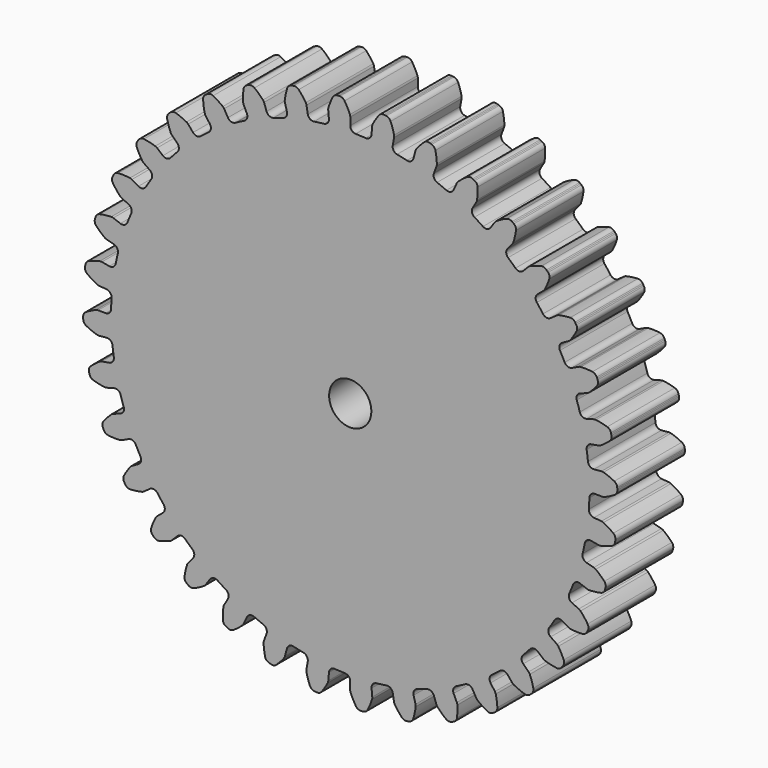
from build123d import *

# Parameters (mm, degrees)
F1_DEPTH = 12.7
F2_R     = 3.175
F3_DEPTH = 12.701


# Not quite as in the source:
# - ends of sketch curves that miss each other by under 0.0002 mm in the source are joined


with BuildPart() as f1:
    # F0 (on Front) → F1 (new body)
    with BuildSketch(Plane.XZ):
        with BuildLine():
            ThreePointArc((-3.2109370393, 36.662551447), (-3.393615267, 36.0650718095), (-3.9425466273, 35.7666968543))
            ThreePointArc((-3.9425466273, 35.7666968543), (-4.6967674834, 35.6754909284), (-5.4488947177, 35.568382366))
            ThreePointArc((-5.4488947177, 35.568382366), (-6.0563468164, 35.7145165506), (-6.3874395437, 36.2443569587))
            Line((-6.3874395437, 36.2443569587), (-6.5805401603, 37.3664180659))
            ThreePointArc((-6.5805401603, 37.3664180659), (-6.6228583498, 37.5208029851), (-6.6941779071, 37.6641175104))
            ThreePointArc((-6.6941779071, 37.6641175104), (-7.1901089353, 38.3817855666), (-7.7496189767, 39.0510714078))
            ThreePointArc((-7.7496189767, 39.0510714078), (-8.1067459622, 39.2794815465), (-8.5301465281, 39.3005252169))
            Line((-8.5301465281, 39.3005252169), (-8.7037167329, 39.2635272434))
            Line((-8.7037167329, 39.2635272434), (-8.7052373822, 39.2631901235))
            Line((-8.7052373822, 39.2631901235), (-8.8781814297, 39.2233677368))
            ThreePointArc((-8.8781814297, 39.2233677368), (-9.2530192202, 39.0253588833), (-9.4801558924, 38.6674206101))
            ThreePointArc((-9.4801558924, 38.6674206101), (-9.704391781, 37.8243824794), (-9.8505583073, 36.9643648225))
            ThreePointArc((-9.8505583073, 36.9643648225), (-9.8546284418, 36.8043368048), (-9.8277358603, 36.6465321107))
            Line((-9.8277358603, 36.6465321107), (-9.5285409381, 35.5479915448))
            ThreePointArc((-9.5285409381, 35.5479915448), (-9.6046926228, 34.9278672241), (-10.0934722151, 34.5387043246))
            ThreePointArc((-10.0934722151, 34.5387043246), (-10.8203970188, 34.3179149444), (-11.5424985437, 34.0818280781))
            ThreePointArc((-11.5424985437, 34.0818280781), (-12.166098015, 34.1202592061), (-12.5841665211, 34.5845564992))
            Line((-12.5841665211, 34.5845564992), (-12.9691773719, 35.6560394067))
            ThreePointArc((-12.9691773719, 35.6560394067), (-13.037661313, 35.8007303955), (-13.1327836721, 35.9294831401))
            ThreePointArc((-13.1327836721, 35.9294831401), (-13.7458021437, 36.5501306866), (-14.413032237, 37.1120906729))
            ThreePointArc((-14.413032237, 37.1120906729), (-14.8043966655, 37.2750162981), (-15.2250190205, 37.2222175312))
            Line((-15.2250190205, 37.2222175312), (-15.3895276731, 37.1556414903))
            Line((-15.3895276731, 37.1556414903), (-15.3909666802, 37.1550454341))
            Line((-15.3909666802, 37.1550454341), (-15.5543682341, 37.0857966202))
            ThreePointArc((-15.5543682341, 37.0857966202), (-15.8891275197, 36.8257060668), (-16.0506581466, 36.4337638111))
            ThreePointArc((-16.0506581466, 36.4337638111), (-16.1250953531, 35.5645951705), (-16.1197007825, 34.6922615633))
            ThreePointArc((-16.1197007825, 34.6922615633), (-16.0959205089, 34.5339579593), (-16.0420339886, 34.3832205209))
            Line((-16.0420339886, 34.3832205209), (-15.5566249422, 33.3533239076))
            ThreePointArc((-15.5566249422, 33.3533239076), (-15.5239362535, 32.7293970675), (-15.9377127572, 32.2612707414))
            ThreePointArc((-15.9377127572, 32.2612707414), (-16.6152542662, 31.9176064805), (-17.2853893923, 31.5597146903))
            ThreePointArc((-17.2853893923, 31.5597146903), (-17.9061884817, 31.4892750513), (-18.3985299667, 31.873921791))
            Line((-18.3985299667, 31.873921791), (-18.9637526919, 32.862270033))
            ThreePointArc((-18.9637526919, 32.862270033), (-19.0563215345, 32.992870729), (-19.1723564507, 33.1031496058))
            ThreePointArc((-19.1723564507, 33.1031496058), (-19.8838361097, 33.607918581), (-20.6385128062, 34.0454778426))
            ThreePointArc((-20.6385128062, 34.0454778426), (-21.0522232676, 34.1379685416), (-21.4572870141, 34.0129316012))
            Line((-21.4572870141, 34.0129316012), (-21.6077356025, 33.9188003722))
            Line((-21.6077356025, 33.9188003722), (-21.6090492437, 33.9179634904))
            Line((-21.6090492437, 33.9179634904), (-21.7579434305, 33.8213923396))
            ThreePointArc((-21.7579434305, 33.8213923396), (-22.0424527198, 33.5071228062), (-22.1334692751, 33.0930855351))
            ThreePointArc((-22.1334692751, 33.0930855351), (-22.0558460626, 32.2241956338), (-21.8990543065, 31.3660514916))
            ThreePointArc((-21.8990543065, 31.3660514916), (-21.8481461763, 31.2142822763), (-21.7689030319, 31.0751921743))
            Line((-21.7689030319, 31.0751921743), (-21.1120287695, 30.145232401))
            ThreePointArc((-21.1120287695, 30.145232401), (-20.9714929366, 29.5364607428), (-21.297693962, 29.0035947717))
            ThreePointArc((-21.297693962, 29.0035947717), (-21.9052654205, 28.5474976948), (-22.5030724311, 28.0786753416))
            ThreePointArc((-22.5030724311, 28.0786753416), (-23.1022084724, 27.9015052085), (-23.6538633894, 28.1948140982))
            Line((-23.6538633894, 28.1948140982), (-24.3821239824, 29.0699972134))
            ThreePointArc((-24.3821239824, 29.0699972134), (-24.4959650692, 29.1825393805), (-24.6293868802, 29.2709936216))
            ThreePointArc((-24.6293868802, 29.2709936216), (-25.4177097773, 29.6445468757), (-26.2369026074, 29.9444103958))
            ThreePointArc((-26.2369026074, 29.9444103958), (-26.6603887185, 29.9636558856), (-27.0375861998, 29.7701799558))
            Line((-27.0375861998, 29.7701799558), (-27.1694034197, 29.6513536685))
            Line((-27.1694034197, 29.6513536685), (-27.1705517807, 29.6503013895))
            Line((-27.1705517807, 29.6503013895), (-27.3004145259, 29.5293421672))
            ThreePointArc((-27.3004145259, 29.5293421672), (-27.526029148, 29.1704425746), (-27.5437661397, 28.746890601))
            ThreePointArc((-27.5437661397, 28.746890601), (-27.3164410503, 27.9046802191), (-27.0130161468, 27.0867998174))
            ThreePointArc((-27.0130161468, 27.0867998174), (-26.9365269778, 26.9461764215), (-26.8343349721, 26.8229598383))
            Line((-26.8343349721, 26.8229598383), (-26.0259542858, 26.0211932622))
            ThreePointArc((-26.0259542858, 26.0211932622), (-25.7818414189, 25.4460740047), (-26.0105555129, 24.8646592514))
            ThreePointArc((-26.0105555129, 24.8646592514), (-26.5296961696, 24.3099876374), (-27.0370110011, 23.7444796512))
            ThreePointArc((-27.0370110011, 23.7444796512), (-27.596279549, 23.4659622487), (-28.1904861423, 23.6590212463))
            Line((-28.1904861423, 23.6590212463), (-29.0596567737, 24.3944472386))
            ThreePointArc((-29.0596567737, 24.3944472386), (-29.1913111008, 24.4855113401), (-29.3380658525, 24.5494533081))
            ThreePointArc((-29.3380658525, 24.5494533081), (-30.1792791952, 24.7804406144), (-31.0380973993, 24.9334971918))
            ThreePointArc((-31.0380973993, 24.9334971918), (-31.4584917491, 24.8789127079), (-31.7963620104, 24.622876457))
            Line((-31.7963620104, 24.622876457), (-31.9055426623, 24.4829655879))
            Line((-31.9055426623, 24.4829655879), (-31.9064908509, 24.4817298846))
            Line((-31.9064908509, 24.4817298846), (-32.0133763406, 24.3400578756))
            ThreePointArc((-32.0133763406, 24.3400578756), (-32.1732411094, 23.9474332063), (-32.117159608, 23.5272359426))
            ThreePointArc((-32.117159608, 23.5272359426), (-31.7470397994, 22.7372952164), (-31.3062011607, 21.9845294373))
            ThreePointArc((-31.3062011607, 21.9845294373), (-31.2064550377, 21.8593246316), (-31.084419223, 21.7557254407))
            Line((-31.084419223, 21.7557254407), (-30.1490943509, 21.1065133335))
            ThreePointArc((-30.1490943509, 21.1065133335), (-29.808821696, 20.5825211842), (-29.9330994966, 19.9702236418))
            ThreePointArc((-29.9330994966, 19.9702236418), (-30.3480355252, 19.333830907), (-30.7494436732, 18.6888199618))
            ThreePointArc((-30.7494436732, 18.6888199618), (-31.2518516358, 18.3174179003), (-31.870555239, 18.4043610059))
            Line((-31.870555239, 18.4043610059), (-32.8542265987, 18.9776843286))
            ThreePointArc((-32.8542265987, 18.9776843286), (-32.9996939161, 19.0445034278), (-33.1553225396, 19.0819902785))
            ThreePointArc((-33.1553225396, 19.0819902785), (-34.0238664862, 19.1633932046), (-34.8962153078, 19.1649922926))
            ThreePointArc((-34.8962153078, 19.1649922926), (-35.3007444267, 19.0382363568), (-35.5890214511, 18.7274193167))
            Line((-35.5890214511, 18.7274193167), (-35.6722481362, 18.5706749869))
            Line((-35.6722481362, 18.5706749869), (-35.6729673419, 18.5692934055))
            Line((-35.6729673419, 18.5692934055), (-35.7536279147, 18.4112132422))
            ThreePointArc((-35.7536279147, 18.4112132422), (-35.8428854202, 17.9967931981), (-35.7146894336, 17.5927181255))
            ThreePointArc((-35.7146894336, 17.5927181255), (-35.2130208091, 16.8790490041), (-34.6481630941, 16.2142702549))
            ThreePointArc((-34.6481630941, 16.2142702549), (-34.5281907524, 16.108288324), (-34.3900191252, 16.0274543345))
            Line((-34.3900191252, 16.0274543345), (-33.3561694403, 15.5505226775))
            ThreePointArc((-33.3561694403, 15.5505226775), (-32.9300760098, 15.0935788729), (-32.9461413989, 14.4690028923))
            ThreePointArc((-32.9461413989, 14.4690028923), (-33.2442651782, 13.7702255079), (-33.5275700593, 13.0653099349))
            ThreePointArc((-33.5275700593, 13.0653099349), (-33.9578520249, 12.6123080781), (-34.5822536419, 12.5904935694))
            Line((-34.5822536419, 12.5904935694), (-35.6505373737, 12.9842940835))
            ThreePointArc((-35.6505373737, 12.9842940835), (-35.8053977304, 13.0248379159), (-35.9651715287, 13.0347306302))
            ThreePointArc((-35.9651715287, 13.0347306302), (-36.834655811, 12.9640757894), (-37.6940293725, 12.8141688005))
            ThreePointArc((-37.6940293725, 12.8141688005), (-38.0704018478, 12.6190928279), (-38.3003264839, 12.2629390171))
            Line((-38.3003264839, 12.2629390171), (-38.3550704014, 12.0941238237))
            Line((-38.3550704014, 12.0941238237), (-38.3555387717, 12.0926383428))
            Line((-38.3555387717, 12.0926383428), (-38.4075235969, 11.9229532109))
            ThreePointArc((-38.4075235969, 11.9229532109), (-38.4234617948, 11.4993297353), (-38.2270464933, 11.1236544704))
            ThreePointArc((-38.2270464933, 11.1236544704), (-37.609072, 10.5079414291), (-36.9373581246, 9.9513486757))
            ThreePointArc((-36.9373581246, 9.9513486757), (-36.8008048633, 9.867809827), (-36.6506956986, 9.8121971386))
            Line((-36.6506956986, 9.8121971386), (-35.5497342003, 9.522037259))
            ThreePointArc((-35.5497342003, 9.522037259), (-35.0507666275, 9.1460258052), (-34.9581314664, 8.5281488117))
            ThreePointArc((-34.9581314664, 8.5281488117), (-35.1303846562, 7.7882187749), (-35.2869781949, 7.044817077))
            ThreePointArc((-35.2869781949, 7.044817077), (-35.6320602637, 6.5239796571), (-36.2431877675, 6.3940703568))
            Line((-36.2431877675, 6.3940703568), (-37.3636246105, 6.5963826331))
            ThreePointArc((-37.3636246105, 6.5963826331), (-37.5231726531, 6.6094192948), (-37.6822369802, 6.5914172876))
            ThreePointArc((-37.6822369802, 6.5914172876), (-38.5262427581, 6.3708514914), (-39.3465294288, 6.0739932736))
            ThreePointArc((-39.3465294288, 6.0739932736), (-39.6833093734, 5.816524549), (-39.8478954775, 5.4258555208))
            Line((-39.8478954775, 5.4258555208), (-39.8724932611, 5.2500988279))
            Line((-39.8724932611, 5.2500988279), (-39.8726965647, 5.2485545832))
            Line((-39.8726965647, 5.2485545832), (-39.8944261097, 5.0724202796))
            ThreePointArc((-39.8944261097, 5.0724202796), (-39.836560726, 4.6524649574), (-39.5778940892, 4.3166042031))
            ThreePointArc((-39.5778940892, 4.3166042031), (-38.8623905695, 3.817555371), (-38.1042302198, 3.3860604026))
            ThreePointArc((-38.1042302198, 3.3860604026), (-37.9552451405, 3.3275029217), (-37.7977594293, 3.2988012979))
            Line((-37.7977594293, 3.2988012979), (-36.6631382757, 3.2042295567))
            ThreePointArc((-36.6631382757, 3.2042295567), (-36.1064574377, 2.9205753715), (-35.907936399, 2.3281712448))
            ThreePointArc((-35.907936399, 2.3281712448), (-35.9490851733, 1.5695709554), (-35.9742093542, 0.8102710171))
            ThreePointArc((-35.9742093542, 0.8102710171), (-36.2236063821, 0.2374234155), (-36.8028909726, 0.003366552))
            Line((-36.8028909726, 0.003366552), (-37.9414370205, 0.0080434342))
            ThreePointArc((-37.9414370205, 0.0080434342), (-38.1008249623, -0.0068231871), (-38.2543467292, -0.0521729338))
            ThreePointArc((-38.2543467292, -0.0521729338), (-39.0472293143, -0.4159479052), (-39.8035050988, -0.8507374652))
            ThreePointArc((-39.8035050988, -0.8507374652), (-40.0904596244, -1.162775885), (-40.1847063309, -1.5760898499))
            Line((-40.1847063309, -1.5760898499), (-40.1784105895, -1.753447764))
            Line((-40.1784105895, -1.753447764), (-40.1783426492, -1.7550038515))
            Line((-40.1783426492, -1.7550038515), (-40.1691566727, -1.9322355751))
            ThreePointArc((-40.1691566727, -1.9322355751), (-40.0392459178, -2.3357626139), (-39.7261874005, -2.6216038985))
            ThreePointArc((-39.7261874005, -2.6216038985), (-38.9348950667, -2.9888251752), (-38.1133245614, -3.2821116025))
            ThreePointArc((-38.1133245614, -3.2821116025), (-37.9564345003, -3.3139084761), (-37.7963573663, -3.314826951))
            Line((-37.7963573663, -3.314826951), (-36.662551447, -3.2109370393))
            ThreePointArc((-36.662551447, -3.2109370393), (-36.0650718095, -3.393615267), (-35.7666968543, -3.9425466273))
            ThreePointArc((-35.7666968543, -3.9425466273), (-35.6754909284, -4.6967674834), (-35.568382366, -5.4488947177))
            ThreePointArc((-35.568382366, -5.4488947177), (-35.7145165506, -6.0563468164), (-36.2443569587, -6.3874395437))
            Line((-36.2443569587, -6.3874395437), (-37.3664180659, -6.5805401603))
            ThreePointArc((-37.3664180659, -6.5805401603), (-37.5208029851, -6.6228583498), (-37.6641175104, -6.6941779071))
            ThreePointArc((-37.6641175104, -6.6941779071), (-38.3817855666, -7.1901089353), (-39.0510714078, -7.7496189767))
            ThreePointArc((-39.0510714078, -7.7496189767), (-39.2794815465, -8.1067459622), (-39.3005252169, -8.5301465281))
            Line((-39.3005252169, -8.5301465281), (-39.2635272434, -8.7037167329))
            Line((-39.2635272434, -8.7037167329), (-39.2631901235, -8.7052373822))
            Line((-39.2631901235, -8.7052373822), (-39.2233677368, -8.8781814297))
            ThreePointArc((-39.2233677368, -8.8781814297), (-39.0253588833, -9.2530192202), (-38.6674206101, -9.4801558924))
            ThreePointArc((-38.6674206101, -9.4801558924), (-37.8243824794, -9.704391781), (-36.9643648225, -9.8505583073))
            ThreePointArc((-36.9643648225, -9.8505583073), (-36.8043368048, -9.8546284418), (-36.6465321107, -9.8277358603))
            Line((-36.6465321107, -9.8277358603), (-35.5479915448, -9.5285409381))
            ThreePointArc((-35.5479915448, -9.5285409381), (-34.9278672241, -9.6046926228), (-34.5387043246, -10.0934722151))
            ThreePointArc((-34.5387043246, -10.0934722151), (-34.3179149444, -10.8203970188), (-34.0818280781, -11.5424985437))
            ThreePointArc((-34.0818280781, -11.5424985437), (-34.1202592061, -12.166098015), (-34.5845564992, -12.5841665211))
            Line((-34.5845564992, -12.5841665211), (-35.6560394067, -12.9691773719))
            ThreePointArc((-35.6560394067, -12.9691773719), (-35.8007303955, -13.037661313), (-35.9294831401, -13.1327836721))
            ThreePointArc((-35.9294831401, -13.1327836721), (-36.5501306866, -13.7458021437), (-37.1120906729, -14.413032237))
            ThreePointArc((-37.1120906729, -14.413032237), (-37.2750162981, -14.8043966655), (-37.2222175312, -15.2250190205))
            Line((-37.2222175312, -15.2250190205), (-37.1556414903, -15.3895276731))
            Line((-37.1556414903, -15.3895276731), (-37.1550454341, -15.3909666802))
            Line((-37.1550454341, -15.3909666802), (-37.0857966202, -15.5543682341))
            ThreePointArc((-37.0857966202, -15.5543682341), (-36.8257060668, -15.8891275197), (-36.4337638111, -16.0506581466))
            ThreePointArc((-36.4337638111, -16.0506581466), (-35.5645951705, -16.1250953531), (-34.6922615633, -16.1197007825))
            ThreePointArc((-34.6922615633, -16.1197007825), (-34.5339579593, -16.0959205089), (-34.3832205209, -16.0420339886))
            Line((-34.3832205209, -16.0420339886), (-33.3533239076, -15.5566249422))
            ThreePointArc((-33.3533239076, -15.5566249422), (-32.7293970675, -15.5239362535), (-32.2612707414, -15.9377127572))
            ThreePointArc((-32.2612707414, -15.9377127572), (-31.9176064805, -16.6152542662), (-31.5597146903, -17.2853893923))
            ThreePointArc((-31.5597146903, -17.2853893923), (-31.4892750513, -17.9061884817), (-31.873921791, -18.3985299667))
            Line((-31.873921791, -18.3985299667), (-32.862270033, -18.9637526919))
            ThreePointArc((-32.862270033, -18.9637526919), (-32.992870729, -19.0563215345), (-33.1031496058, -19.1723564507))
            ThreePointArc((-33.1031496058, -19.1723564507), (-33.607918581, -19.8838361097), (-34.0454778426, -20.6385128062))
            ThreePointArc((-34.0454778426, -20.6385128062), (-34.1379685416, -21.0522232676), (-34.0129316012, -21.4572870141))
            Line((-34.0129316012, -21.4572870141), (-33.9188003722, -21.6077356025))
            Line((-33.9188003722, -21.6077356025), (-33.9179634904, -21.6090492437))
            Line((-33.9179634904, -21.6090492437), (-33.8213923396, -21.7579434305))
            ThreePointArc((-33.8213923396, -21.7579434305), (-33.5071228062, -22.0424527198), (-33.0930855351, -22.1334692751))
            ThreePointArc((-33.0930855351, -22.1334692751), (-32.2241956338, -22.0558460626), (-31.3660514916, -21.8990543065))
            ThreePointArc((-31.3660514916, -21.8990543065), (-31.2142822763, -21.8481461763), (-31.0751921743, -21.7689030319))
            Line((-31.0751921743, -21.7689030319), (-30.145232401, -21.1120287695))
            ThreePointArc((-30.145232401, -21.1120287695), (-29.5364607428, -20.9714929366), (-29.0035947717, -21.297693962))
            ThreePointArc((-29.0035947717, -21.297693962), (-28.5474976948, -21.9052654205), (-28.0786753416, -22.5030724311))
            ThreePointArc((-28.0786753416, -22.5030724311), (-27.9015052085, -23.1022084724), (-28.1948140982, -23.6538633894))
            Line((-28.1948140982, -23.6538633894), (-29.0699972134, -24.3821239824))
            ThreePointArc((-29.0699972134, -24.3821239824), (-29.1825393805, -24.4959650692), (-29.2709936216, -24.6293868802))
            ThreePointArc((-29.2709936216, -24.6293868802), (-29.6445468757, -25.4177097773), (-29.9444103958, -26.2369026074))
            ThreePointArc((-29.9444103958, -26.2369026074), (-29.9636558856, -26.6603887185), (-29.7701799558, -27.0375861998))
            Line((-29.7701799558, -27.0375861998), (-29.6513536685, -27.1694034197))
            Line((-29.6513536685, -27.1694034197), (-29.6503013895, -27.1705517807))
            Line((-29.6503013895, -27.1705517807), (-29.5293421672, -27.3004145259))
            ThreePointArc((-29.5293421672, -27.3004145259), (-29.1704425746, -27.526029148), (-28.746890601, -27.5437661397))
            ThreePointArc((-28.746890601, -27.5437661397), (-27.9046802191, -27.3164410503), (-27.0867998174, -27.0130161468))
            ThreePointArc((-27.0867998174, -27.0130161468), (-26.9461764215, -26.9365269778), (-26.8229598383, -26.8343349721))
            Line((-26.8229598383, -26.8343349721), (-26.0211932622, -26.0259542858))
            ThreePointArc((-26.0211932622, -26.0259542858), (-25.4460740047, -25.7818414189), (-24.8646592514, -26.0105555129))
            ThreePointArc((-24.8646592514, -26.0105555129), (-24.3099876374, -26.5296961696), (-23.7444796512, -27.0370110011))
            ThreePointArc((-23.7444796512, -27.0370110011), (-23.4659622487, -27.596279549), (-23.6590212463, -28.1904861423))
            Line((-23.6590212463, -28.1904861423), (-24.3944472386, -29.0596567737))
            ThreePointArc((-24.3944472386, -29.0596567737), (-24.4855113401, -29.1913111008), (-24.5494533081, -29.3380658525))
            ThreePointArc((-24.5494533081, -29.3380658525), (-24.7804406144, -30.1792791952), (-24.9334971918, -31.0380973993))
            ThreePointArc((-24.9334971918, -31.0380973993), (-24.8789127079, -31.4584917491), (-24.622876457, -31.7963620104))
            Line((-24.622876457, -31.7963620104), (-24.4829655879, -31.9055426623))
            Line((-24.4829655879, -31.9055426623), (-24.4817298846, -31.9064908509))
            Line((-24.4817298846, -31.9064908509), (-24.3400578756, -32.0133763406))
            ThreePointArc((-24.3400578756, -32.0133763406), (-23.9474332063, -32.1732411094), (-23.5272359426, -32.117159608))
            ThreePointArc((-23.5272359426, -32.117159608), (-22.7372952164, -31.7470397994), (-21.9845294373, -31.3062011607))
            ThreePointArc((-21.9845294373, -31.3062011607), (-21.8593246316, -31.2064550377), (-21.7557254407, -31.084419223))
            Line((-21.7557254407, -31.084419223), (-21.1065133335, -30.1490943509))
            ThreePointArc((-21.1065133335, -30.1490943509), (-20.5825211842, -29.808821696), (-19.9702236418, -29.9330994966))
            ThreePointArc((-19.9702236418, -29.9330994966), (-19.333830907, -30.3480355252), (-18.6888199618, -30.7494436732))
            ThreePointArc((-18.6888199618, -30.7494436732), (-18.3174179003, -31.2518516358), (-18.4043610059, -31.870555239))
            Line((-18.4043610059, -31.870555239), (-18.9776843286, -32.8542265987))
            ThreePointArc((-18.9776843286, -32.8542265987), (-19.0445034278, -32.9996939161), (-19.0819902785, -33.1553225396))
            ThreePointArc((-19.0819902785, -33.1553225396), (-19.1633932046, -34.0238664862), (-19.1649922926, -34.8962153078))
            ThreePointArc((-19.1649922926, -34.8962153078), (-19.0382363568, -35.3007444267), (-18.7274193167, -35.5890214511))
            Line((-18.7274193167, -35.5890214511), (-18.5706749869, -35.6722481362))
            Line((-18.5706749869, -35.6722481362), (-18.5692934055, -35.6729673419))
            Line((-18.5692934055, -35.6729673419), (-18.4112132422, -35.7536279147))
            ThreePointArc((-18.4112132422, -35.7536279147), (-17.9967931981, -35.8428854202), (-17.5927181255, -35.7146894336))
            ThreePointArc((-17.5927181255, -35.7146894336), (-16.8790490041, -35.2130208091), (-16.2142702549, -34.6481630941))
            ThreePointArc((-16.2142702549, -34.6481630941), (-16.108288324, -34.5281907524), (-16.0274543345, -34.3900191252))
            Line((-16.0274543345, -34.3900191252), (-15.5505226775, -33.3561694403))
            ThreePointArc((-15.5505226775, -33.3561694403), (-15.0935788729, -32.9300760098), (-14.4690028923, -32.9461413989))
            ThreePointArc((-14.4690028923, -32.9461413989), (-13.7702255079, -33.2442651782), (-13.0653099349, -33.5275700593))
            ThreePointArc((-13.0653099349, -33.5275700593), (-12.6123080781, -33.9578520249), (-12.5904935694, -34.5822536419))
            Line((-12.5904935694, -34.5822536419), (-12.9842940835, -35.6505373737))
            ThreePointArc((-12.9842940835, -35.6505373737), (-13.0248379159, -35.8053977304), (-13.0347306302, -35.9651715287))
            ThreePointArc((-13.0347306302, -35.9651715287), (-12.9640757894, -36.834655811), (-12.8141688005, -37.6940293725))
            ThreePointArc((-12.8141688005, -37.6940293725), (-12.6190928279, -38.0704018478), (-12.2629390171, -38.3003264839))
            Line((-12.2629390171, -38.3003264839), (-12.0941238237, -38.3550704014))
            Line((-12.0941238237, -38.3550704014), (-12.0926383428, -38.3555387717))
            Line((-12.0926383428, -38.3555387717), (-11.9229532109, -38.4075235969))
            ThreePointArc((-11.9229532109, -38.4075235969), (-11.4993297353, -38.4234617948), (-11.1236544704, -38.2270464933))
            ThreePointArc((-11.1236544704, -38.2270464933), (-10.5079414291, -37.609072), (-9.9513486757, -36.9373581246))
            ThreePointArc((-9.9513486757, -36.9373581246), (-9.867809827, -36.8008048633), (-9.8121971386, -36.6506956986))
            Line((-9.8121971386, -36.6506956986), (-9.522037259, -35.5497342003))
            ThreePointArc((-9.522037259, -35.5497342003), (-9.1460258052, -35.0507666275), (-8.5281488117, -34.9581314664))
            ThreePointArc((-8.5281488117, -34.9581314664), (-7.7882187749, -35.1303846562), (-7.044817077, -35.2869781949))
            ThreePointArc((-7.044817077, -35.2869781949), (-6.5239796571, -35.6320602637), (-6.3940703568, -36.2431877675))
            Line((-6.3940703568, -36.2431877675), (-6.5963826331, -37.3636246105))
            ThreePointArc((-6.5963826331, -37.3636246105), (-6.6094192948, -37.5231726531), (-6.5914172876, -37.6822369802))
            ThreePointArc((-6.5914172876, -37.6822369802), (-6.3708514914, -38.5262427581), (-6.0739932736, -39.3465294288))
            ThreePointArc((-6.0739932736, -39.3465294288), (-5.816524549, -39.6833093734), (-5.4258555208, -39.8478954775))
            Line((-5.4258555208, -39.8478954775), (-5.2500988279, -39.8724932611))
            Line((-5.2500988279, -39.8724932611), (-5.2485545832, -39.8726965647))
            Line((-5.2485545832, -39.8726965647), (-5.0724202796, -39.8944261097))
            ThreePointArc((-5.0724202796, -39.8944261097), (-4.6524649574, -39.836560726), (-4.3166042031, -39.5778940892))
            ThreePointArc((-4.3166042031, -39.5778940892), (-3.817555371, -38.8623905695), (-3.3860604026, -38.1042302198))
            ThreePointArc((-3.3860604026, -38.1042302198), (-3.3275029217, -37.9552451405), (-3.2988012979, -37.7977594293))
            Line((-3.2988012979, -37.7977594293), (-3.2042295567, -36.6631382757))
            ThreePointArc((-3.2042295567, -36.6631382757), (-2.9205753715, -36.1064574377), (-2.3281712448, -35.907936399))
            ThreePointArc((-2.3281712448, -35.907936399), (-1.5695709554, -35.9490851733), (-0.8102710171, -35.9742093542))
            ThreePointArc((-0.8102710171, -35.9742093542), (-0.2374234155, -36.2236063821), (-0.003366552, -36.8028909726))
            Line((-0.003366552, -36.8028909726), (-0.0080434342, -37.9414370205))
            ThreePointArc((-0.0080434342, -37.9414370205), (0.0068231871, -38.1008249623), (0.0521729338, -38.2543467292))
            ThreePointArc((0.0521729338, -38.2543467292), (0.4159479052, -39.0472293143), (0.8507374652, -39.8035050988))
            ThreePointArc((0.8507374652, -39.8035050988), (1.162775885, -40.0904596244), (1.5760898499, -40.1847063309))
            Line((1.5760898499, -40.1847063309), (1.753447764, -40.1784105895))
            Line((1.753447764, -40.1784105895), (1.7550038515, -40.1783426492))
            Line((1.7550038515, -40.1783426492), (1.9322355751, -40.1691566727))
            ThreePointArc((1.9322355751, -40.1691566727), (2.3357626139, -40.0392459178), (2.6216038985, -39.7261874005))
            ThreePointArc((2.6216038985, -39.7261874005), (2.9888251752, -38.9348950667), (3.2821116025, -38.1133245614))
            ThreePointArc((3.2821116025, -38.1133245614), (3.3139084761, -37.9564345003), (3.314826951, -37.7963573663))
            Line((3.314826951, -37.7963573663), (3.2109370393, -36.662551447))
            ThreePointArc((3.2109370393, -36.662551447), (3.393615267, -36.0650718095), (3.9425466273, -35.7666968543))
            ThreePointArc((3.9425466273, -35.7666968543), (4.6967674834, -35.6754909284), (5.4488947177, -35.568382366))
            ThreePointArc((5.4488947177, -35.568382366), (6.0563468164, -35.7145165506), (6.3874395437, -36.2443569587))
            Line((6.3874395437, -36.2443569587), (6.5805401603, -37.3664180659))
            ThreePointArc((6.5805401603, -37.3664180659), (6.6228583498, -37.5208029851), (6.6941779071, -37.6641175104))
            ThreePointArc((6.6941779071, -37.6641175104), (7.1901089353, -38.3817855666), (7.7496189767, -39.0510714078))
            ThreePointArc((7.7496189767, -39.0510714078), (8.1067459622, -39.2794815465), (8.5301465281, -39.3005252169))
            Line((8.5301465281, -39.3005252169), (8.7037167329, -39.2635272434))
            Line((8.7037167329, -39.2635272434), (8.7052373822, -39.2631901235))
            Line((8.7052373822, -39.2631901235), (8.8781814297, -39.2233677368))
            ThreePointArc((8.8781814297, -39.2233677368), (9.2530192202, -39.0253588833), (9.4801558924, -38.6674206101))
            ThreePointArc((9.4801558924, -38.6674206101), (9.704391781, -37.8243824794), (9.8505583073, -36.9643648225))
            ThreePointArc((9.8505583073, -36.9643648225), (9.8546284418, -36.8043368048), (9.8277358603, -36.6465321107))
            Line((9.8277358603, -36.6465321107), (9.5285409381, -35.5479915448))
            ThreePointArc((9.5285409381, -35.5479915448), (9.6046926228, -34.9278672241), (10.0934722151, -34.5387043246))
            ThreePointArc((10.0934722151, -34.5387043246), (10.8203970188, -34.3179149444), (11.5424985437, -34.0818280781))
            ThreePointArc((11.5424985437, -34.0818280781), (12.166098015, -34.1202592061), (12.5841665211, -34.5845564992))
            Line((12.5841665211, -34.5845564992), (12.9691773719, -35.6560394067))
            ThreePointArc((12.9691773719, -35.6560394067), (13.037661313, -35.8007303955), (13.1327836721, -35.9294831401))
            ThreePointArc((13.1327836721, -35.9294831401), (13.7458021437, -36.5501306866), (14.413032237, -37.1120906729))
            ThreePointArc((14.413032237, -37.1120906729), (14.8043966655, -37.2750162981), (15.2250190205, -37.2222175312))
            Line((15.2250190205, -37.2222175312), (15.3895276731, -37.1556414903))
            Line((15.3895276731, -37.1556414903), (15.3909666802, -37.1550454341))
            Line((15.3909666802, -37.1550454341), (15.5543682341, -37.0857966202))
            ThreePointArc((15.5543682341, -37.0857966202), (15.8891275197, -36.8257060668), (16.0506581466, -36.4337638111))
            ThreePointArc((16.0506581466, -36.4337638111), (16.1250953531, -35.5645951705), (16.1197007825, -34.6922615633))
            ThreePointArc((16.1197007825, -34.6922615633), (16.0959205089, -34.5339579593), (16.0420339886, -34.3832205209))
            Line((16.0420339886, -34.3832205209), (15.5566249422, -33.3533239076))
            ThreePointArc((15.5566249422, -33.3533239076), (15.5239362535, -32.7293970675), (15.9377127572, -32.2612707414))
            ThreePointArc((15.9377127572, -32.2612707414), (16.6152542662, -31.9176064805), (17.2853893923, -31.5597146903))
            ThreePointArc((17.2853893923, -31.5597146903), (17.9061884817, -31.4892750513), (18.3985299667, -31.873921791))
            Line((18.3985299667, -31.873921791), (18.9637526919, -32.862270033))
            ThreePointArc((18.9637526919, -32.862270033), (19.0563215345, -32.992870729), (19.1723564507, -33.1031496058))
            ThreePointArc((19.1723564507, -33.1031496058), (19.8838361097, -33.607918581), (20.6385128062, -34.0454778426))
            ThreePointArc((20.6385128062, -34.0454778426), (21.0522232676, -34.1379685416), (21.4572870141, -34.0129316012))
            Line((21.4572870141, -34.0129316012), (21.6077356025, -33.9188003722))
            Line((21.6077356025, -33.9188003722), (21.6090492437, -33.9179634904))
            Line((21.6090492437, -33.9179634904), (21.7579434305, -33.8213923396))
            ThreePointArc((21.7579434305, -33.8213923396), (22.0424527198, -33.5071228062), (22.1334692751, -33.0930855351))
            ThreePointArc((22.1334692751, -33.0930855351), (22.0558460626, -32.2241956338), (21.8990543065, -31.3660514916))
            ThreePointArc((21.8990543065, -31.3660514916), (21.8481461763, -31.2142822763), (21.7689030319, -31.0751921743))
            Line((21.7689030319, -31.0751921743), (21.1120287695, -30.145232401))
            ThreePointArc((21.1120287695, -30.145232401), (20.9714929366, -29.5364607428), (21.297693962, -29.0035947717))
            ThreePointArc((21.297693962, -29.0035947717), (21.9052654205, -28.5474976948), (22.5030724311, -28.0786753416))
            ThreePointArc((22.5030724311, -28.0786753416), (23.1022084724, -27.9015052085), (23.6538633894, -28.1948140982))
            Line((23.6538633894, -28.1948140982), (24.3821239824, -29.0699972134))
            ThreePointArc((24.3821239824, -29.0699972134), (24.4959650692, -29.1825393805), (24.6293868802, -29.2709936216))
            ThreePointArc((24.6293868802, -29.2709936216), (25.4177097773, -29.6445468757), (26.2369026074, -29.9444103958))
            ThreePointArc((26.2369026074, -29.9444103958), (26.6603887185, -29.9636558856), (27.0375861998, -29.7701799558))
            Line((27.0375861998, -29.7701799558), (27.1694034197, -29.6513536685))
            Line((27.1694034197, -29.6513536685), (27.1705517807, -29.6503013895))
            Line((27.1705517807, -29.6503013895), (27.3004145259, -29.5293421672))
            ThreePointArc((27.3004145259, -29.5293421672), (27.526029148, -29.1704425746), (27.5437661397, -28.746890601))
            ThreePointArc((27.5437661397, -28.746890601), (27.3164410503, -27.9046802191), (27.0130161468, -27.0867998174))
            ThreePointArc((27.0130161468, -27.0867998174), (26.9365269778, -26.9461764215), (26.8343349721, -26.8229598383))
            Line((26.8343349721, -26.8229598383), (26.0259542858, -26.0211932622))
            ThreePointArc((26.0259542858, -26.0211932622), (25.7818414189, -25.4460740047), (26.0105555129, -24.8646592514))
            ThreePointArc((26.0105555129, -24.8646592514), (26.5296961696, -24.3099876374), (27.0370110011, -23.7444796512))
            ThreePointArc((27.0370110011, -23.7444796512), (27.596279549, -23.4659622487), (28.1904861423, -23.6590212463))
            Line((28.1904861423, -23.6590212463), (29.0596567737, -24.3944472386))
            ThreePointArc((29.0596567737, -24.3944472386), (29.1913111008, -24.4855113401), (29.3380658525, -24.5494533081))
            ThreePointArc((29.3380658525, -24.5494533081), (30.1792791952, -24.7804406144), (31.0380973993, -24.9334971918))
            ThreePointArc((31.0380973993, -24.9334971918), (31.4584917491, -24.8789127079), (31.7963620104, -24.622876457))
            Line((31.7963620104, -24.622876457), (31.9055426623, -24.4829655879))
            Line((31.9055426623, -24.4829655879), (31.9064908509, -24.4817298846))
            Line((31.9064908509, -24.4817298846), (32.0133763406, -24.3400578756))
            ThreePointArc((32.0133763406, -24.3400578756), (32.1732411094, -23.9474332063), (32.117159608, -23.5272359426))
            ThreePointArc((32.117159608, -23.5272359426), (31.7470397994, -22.7372952164), (31.3062011607, -21.9845294373))
            ThreePointArc((31.3062011607, -21.9845294373), (31.2064550377, -21.8593246316), (31.084419223, -21.7557254407))
            Line((31.084419223, -21.7557254407), (30.1490943509, -21.1065133335))
            ThreePointArc((30.1490943509, -21.1065133335), (29.808821696, -20.5825211842), (29.9330994966, -19.9702236418))
            ThreePointArc((29.9330994966, -19.9702236418), (30.3480355252, -19.333830907), (30.7494436732, -18.6888199618))
            ThreePointArc((30.7494436732, -18.6888199618), (31.2518516358, -18.3174179003), (31.870555239, -18.4043610059))
            Line((31.870555239, -18.4043610059), (32.8542265987, -18.9776843286))
            ThreePointArc((32.8542265987, -18.9776843286), (32.9996939161, -19.0445034278), (33.1553225396, -19.0819902785))
            ThreePointArc((33.1553225396, -19.0819902785), (34.0238664862, -19.1633932046), (34.8962153078, -19.1649922926))
            ThreePointArc((34.8962153078, -19.1649922926), (35.3007444267, -19.0382363568), (35.5890214511, -18.7274193167))
            Line((35.5890214511, -18.7274193167), (35.6722481362, -18.5706749869))
            Line((35.6722481362, -18.5706749869), (35.6729673419, -18.5692934055))
            Line((35.6729673419, -18.5692934055), (35.7536279147, -18.4112132422))
            ThreePointArc((35.7536279147, -18.4112132422), (35.8428854202, -17.9967931981), (35.7146894336, -17.5927181255))
            ThreePointArc((35.7146894336, -17.5927181255), (35.2130208091, -16.8790490041), (34.6481630941, -16.2142702549))
            ThreePointArc((34.6481630941, -16.2142702549), (34.5281907524, -16.108288324), (34.3900191252, -16.0274543345))
            Line((34.3900191252, -16.0274543345), (33.3561694403, -15.5505226775))
            ThreePointArc((33.3561694403, -15.5505226775), (32.9300760098, -15.0935788729), (32.9461413989, -14.4690028923))
            ThreePointArc((32.9461413989, -14.4690028923), (33.2442651782, -13.7702255079), (33.5275700593, -13.0653099349))
            ThreePointArc((33.5275700593, -13.0653099349), (33.9578520249, -12.6123080781), (34.5822536419, -12.5904935694))
            Line((34.5822536419, -12.5904935694), (35.6505373737, -12.9842940835))
            ThreePointArc((35.6505373737, -12.9842940835), (35.8053977304, -13.0248379159), (35.9651715287, -13.0347306302))
            ThreePointArc((35.9651715287, -13.0347306302), (36.834655811, -12.9640757894), (37.6940293725, -12.8141688005))
            ThreePointArc((37.6940293725, -12.8141688005), (38.0704018478, -12.6190928279), (38.3003264839, -12.2629390171))
            Line((38.3003264839, -12.2629390171), (38.3550704014, -12.0941238237))
            Line((38.3550704014, -12.0941238237), (38.3555387717, -12.0926383428))
            Line((38.3555387717, -12.0926383428), (38.4075235969, -11.9229532109))
            ThreePointArc((38.4075235969, -11.9229532109), (38.4234617948, -11.4993297353), (38.2270464933, -11.1236544704))
            ThreePointArc((38.2270464933, -11.1236544704), (37.609072, -10.5079414291), (36.9373581246, -9.9513486757))
            ThreePointArc((36.9373581246, -9.9513486757), (36.8008048633, -9.867809827), (36.6506956986, -9.8121971386))
            Line((36.6506956986, -9.8121971386), (35.5497342003, -9.522037259))
            ThreePointArc((35.5497342003, -9.522037259), (35.0507666275, -9.1460258052), (34.9581314664, -8.5281488117))
            ThreePointArc((34.9581314664, -8.5281488117), (35.1303846562, -7.7882187749), (35.2869781949, -7.044817077))
            ThreePointArc((35.2869781949, -7.044817077), (35.6320602637, -6.5239796571), (36.2431877675, -6.3940703568))
            Line((36.2431877675, -6.3940703568), (37.3636246105, -6.5963826331))
            ThreePointArc((37.3636246105, -6.5963826331), (37.5231726531, -6.6094192948), (37.6822369802, -6.5914172876))
            ThreePointArc((37.6822369802, -6.5914172876), (38.5262427581, -6.3708514914), (39.3465294288, -6.0739932736))
            ThreePointArc((39.3465294288, -6.0739932736), (39.6833093734, -5.816524549), (39.8478954775, -5.4258555208))
            Line((39.8478954775, -5.4258555208), (39.8724932611, -5.2500988279))
            Line((39.8724932611, -5.2500988279), (39.8726965647, -5.2485545832))
            Line((39.8726965647, -5.2485545832), (39.8944261097, -5.0724202796))
            ThreePointArc((39.8944261097, -5.0724202796), (39.836560726, -4.6524649574), (39.5778940892, -4.3166042031))
            ThreePointArc((39.5778940892, -4.3166042031), (38.8623905695, -3.817555371), (38.1042302198, -3.3860604026))
            ThreePointArc((38.1042302198, -3.3860604026), (37.9552451405, -3.3275029217), (37.7977594293, -3.2988012979))
            Line((37.7977594293, -3.2988012979), (36.6631382757, -3.2042295567))
            ThreePointArc((36.6631382757, -3.2042295567), (36.1064574377, -2.9205753715), (35.907936399, -2.3281712448))
            ThreePointArc((35.907936399, -2.3281712448), (35.9490851733, -1.5695709554), (35.9742093542, -0.8102710171))
            ThreePointArc((35.9742093542, -0.8102710171), (36.2236063821, -0.2374234155), (36.8028909726, -0.003366552))
            Line((36.8028909726, -0.003366552), (37.9414370205, -0.0080434342))
            ThreePointArc((37.9414370205, -0.0080434342), (38.1008249623, 0.0068231871), (38.2543467292, 0.0521729338))
            ThreePointArc((38.2543467292, 0.0521729338), (39.0472293143, 0.4159479052), (39.8035050988, 0.8507374652))
            ThreePointArc((39.8035050988, 0.8507374652), (40.0904596244, 1.162775885), (40.1847063309, 1.5760898499))
            Line((40.1847063309, 1.5760898499), (40.1784105895, 1.753447764))
            Line((40.1784105895, 1.753447764), (40.1783426492, 1.7550038515))
            Line((40.1783426492, 1.7550038515), (40.1691566727, 1.9322355751))
            ThreePointArc((40.1691566727, 1.9322355751), (40.0392459178, 2.3357626139), (39.7261874005, 2.6216038985))
            ThreePointArc((39.7261874005, 2.6216038985), (38.9348950667, 2.9888251752), (38.1133245614, 3.2821116025))
            ThreePointArc((38.1133245614, 3.2821116025), (37.9564345003, 3.3139084761), (37.7963573663, 3.314826951))
            Line((37.7963573663, 3.314826951), (36.662551447, 3.2109370393))
            ThreePointArc((36.662551447, 3.2109370393), (36.0650718095, 3.393615267), (35.7666968543, 3.9425466273))
            ThreePointArc((35.7666968543, 3.9425466273), (35.6754909284, 4.6967674834), (35.568382366, 5.4488947177))
            ThreePointArc((35.568382366, 5.4488947177), (35.7145165506, 6.0563468164), (36.2443569587, 6.3874395437))
            Line((36.2443569587, 6.3874395437), (37.3664180659, 6.5805401603))
            ThreePointArc((37.3664180659, 6.5805401603), (37.5208029851, 6.6228583498), (37.6641175104, 6.6941779071))
            ThreePointArc((37.6641175104, 6.6941779071), (38.3817855666, 7.1901089353), (39.0510714078, 7.7496189767))
            ThreePointArc((39.0510714078, 7.7496189767), (39.2794815465, 8.1067459622), (39.3005252169, 8.5301465281))
            Line((39.3005252169, 8.5301465281), (39.2635272434, 8.7037167329))
            Line((39.2635272434, 8.7037167329), (39.2631901235, 8.7052373822))
            Line((39.2631901235, 8.7052373822), (39.2233677368, 8.8781814297))
            ThreePointArc((39.2233677368, 8.8781814297), (39.0253588833, 9.2530192202), (38.6674206101, 9.4801558924))
            ThreePointArc((38.6674206101, 9.4801558924), (37.8243824794, 9.704391781), (36.9643648225, 9.8505583073))
            ThreePointArc((36.9643648225, 9.8505583073), (36.8043368048, 9.8546284418), (36.6465321107, 9.8277358603))
            Line((36.6465321107, 9.8277358603), (35.5479915448, 9.5285409381))
            ThreePointArc((35.5479915448, 9.5285409381), (34.9278672241, 9.6046926228), (34.5387043246, 10.0934722151))
            ThreePointArc((34.5387043246, 10.0934722151), (34.3179149444, 10.8203970188), (34.0818280781, 11.5424985437))
            ThreePointArc((34.0818280781, 11.5424985437), (34.1202592061, 12.166098015), (34.5845564992, 12.5841665211))
            Line((34.5845564992, 12.5841665211), (35.6560394067, 12.9691773719))
            ThreePointArc((35.6560394067, 12.9691773719), (35.8007303955, 13.037661313), (35.9294831401, 13.1327836721))
            ThreePointArc((35.9294831401, 13.1327836721), (36.5501306866, 13.7458021437), (37.1120906729, 14.413032237))
            ThreePointArc((37.1120906729, 14.413032237), (37.2750162981, 14.8043966655), (37.2222175312, 15.2250190205))
            Line((37.2222175312, 15.2250190205), (37.1556414903, 15.3895276731))
            Line((37.1556414903, 15.3895276731), (37.1550454341, 15.3909666802))
            Line((37.1550454341, 15.3909666802), (37.0857966202, 15.5543682341))
            ThreePointArc((37.0857966202, 15.5543682341), (36.8257060668, 15.8891275197), (36.4337638111, 16.0506581466))
            ThreePointArc((36.4337638111, 16.0506581466), (35.5645951705, 16.1250953531), (34.6922615633, 16.1197007825))
            ThreePointArc((34.6922615633, 16.1197007825), (34.5339579593, 16.0959205089), (34.3832205209, 16.0420339886))
            Line((34.3832205209, 16.0420339886), (33.3533239076, 15.5566249422))
            ThreePointArc((33.3533239076, 15.5566249422), (32.7293970675, 15.5239362535), (32.2612707414, 15.9377127572))
            ThreePointArc((32.2612707414, 15.9377127572), (31.9176064805, 16.6152542662), (31.5597146903, 17.2853893923))
            ThreePointArc((31.5597146903, 17.2853893923), (31.4892750513, 17.9061884817), (31.873921791, 18.3985299667))
            Line((31.873921791, 18.3985299667), (32.862270033, 18.9637526919))
            ThreePointArc((32.862270033, 18.9637526919), (32.992870729, 19.0563215345), (33.1031496058, 19.1723564507))
            ThreePointArc((33.1031496058, 19.1723564507), (33.607918581, 19.8838361097), (34.0454778426, 20.6385128062))
            ThreePointArc((34.0454778426, 20.6385128062), (34.1379685416, 21.0522232676), (34.0129316012, 21.4572870141))
            Line((34.0129316012, 21.4572870141), (33.9188003722, 21.6077356025))
            Line((33.9188003722, 21.6077356025), (33.9179634904, 21.6090492437))
            Line((33.9179634904, 21.6090492437), (33.8213923396, 21.7579434305))
            ThreePointArc((33.8213923396, 21.7579434305), (33.5071228062, 22.0424527198), (33.0930855351, 22.1334692751))
            ThreePointArc((33.0930855351, 22.1334692751), (32.2241956338, 22.0558460626), (31.3660514916, 21.8990543065))
            ThreePointArc((31.3660514916, 21.8990543065), (31.2142822763, 21.8481461763), (31.0751921743, 21.7689030319))
            Line((31.0751921743, 21.7689030319), (30.145232401, 21.1120287695))
            ThreePointArc((30.145232401, 21.1120287695), (29.5364607428, 20.9714929366), (29.0035947717, 21.297693962))
            ThreePointArc((29.0035947717, 21.297693962), (28.5474976948, 21.9052654205), (28.0786753416, 22.5030724311))
            ThreePointArc((28.0786753416, 22.5030724311), (27.9015052085, 23.1022084724), (28.1948140982, 23.6538633894))
            Line((28.1948140982, 23.6538633894), (29.0699972134, 24.3821239824))
            ThreePointArc((29.0699972134, 24.3821239824), (29.1825393805, 24.4959650692), (29.2709936216, 24.6293868802))
            ThreePointArc((29.2709936216, 24.6293868802), (29.6445468757, 25.4177097773), (29.9444103958, 26.2369026074))
            ThreePointArc((29.9444103958, 26.2369026074), (29.9636558856, 26.6603887185), (29.7701799558, 27.0375861998))
            Line((29.7701799558, 27.0375861998), (29.6513536685, 27.1694034197))
            Line((29.6513536685, 27.1694034197), (29.6503013895, 27.1705517807))
            Line((29.6503013895, 27.1705517807), (29.5293421672, 27.3004145259))
            ThreePointArc((29.5293421672, 27.3004145259), (29.1704425746, 27.526029148), (28.746890601, 27.5437661397))
            ThreePointArc((28.746890601, 27.5437661397), (27.9046802191, 27.3164410503), (27.0867998174, 27.0130161468))
            ThreePointArc((27.0867998174, 27.0130161468), (26.9461764215, 26.9365269778), (26.8229598383, 26.8343349721))
            Line((26.8229598383, 26.8343349721), (26.0211932622, 26.0259542858))
            ThreePointArc((26.0211932622, 26.0259542858), (25.4460740047, 25.7818414189), (24.8646592514, 26.0105555129))
            ThreePointArc((24.8646592514, 26.0105555129), (24.3099876374, 26.5296961696), (23.7444796512, 27.0370110011))
            ThreePointArc((23.7444796512, 27.0370110011), (23.4659622487, 27.596279549), (23.6590212463, 28.1904861423))
            Line((23.6590212463, 28.1904861423), (24.3944472386, 29.0596567737))
            ThreePointArc((24.3944472386, 29.0596567737), (24.4855113401, 29.1913111008), (24.5494533081, 29.3380658525))
            ThreePointArc((24.5494533081, 29.3380658525), (24.7804406144, 30.1792791952), (24.9334971918, 31.0380973993))
            ThreePointArc((24.9334971918, 31.0380973993), (24.8789127079, 31.4584917491), (24.622876457, 31.7963620104))
            Line((24.622876457, 31.7963620104), (24.4829655879, 31.9055426623))
            Line((24.4829655879, 31.9055426623), (24.4817298846, 31.9064908509))
            Line((24.4817298846, 31.9064908509), (24.3400578756, 32.0133763406))
            ThreePointArc((24.3400578756, 32.0133763406), (23.9474332063, 32.1732411094), (23.5272359426, 32.117159608))
            ThreePointArc((23.5272359426, 32.117159608), (22.7372952164, 31.7470397994), (21.9845294373, 31.3062011607))
            ThreePointArc((21.9845294373, 31.3062011607), (21.8593246316, 31.2064550377), (21.7557254407, 31.084419223))
            Line((21.7557254407, 31.084419223), (21.1065133335, 30.1490943509))
            ThreePointArc((21.1065133335, 30.1490943509), (20.5825211842, 29.808821696), (19.9702236418, 29.9330994966))
            ThreePointArc((19.9702236418, 29.9330994966), (19.333830907, 30.3480355252), (18.6888199618, 30.7494436732))
            ThreePointArc((18.6888199618, 30.7494436732), (18.3174179003, 31.2518516358), (18.4043610059, 31.870555239))
            Line((18.4043610059, 31.870555239), (18.9776843286, 32.8542265987))
            ThreePointArc((18.9776843286, 32.8542265987), (19.0445034278, 32.9996939161), (19.0819902785, 33.1553225396))
            ThreePointArc((19.0819902785, 33.1553225396), (19.1633932046, 34.0238664862), (19.1649922926, 34.8962153078))
            ThreePointArc((19.1649922926, 34.8962153078), (19.0382363568, 35.3007444267), (18.7274193167, 35.5890214511))
            Line((18.7274193167, 35.5890214511), (18.5706749869, 35.6722481362))
            Line((18.5706749869, 35.6722481362), (18.5692934055, 35.6729673419))
            Line((18.5692934055, 35.6729673419), (18.4112132422, 35.7536279147))
            ThreePointArc((18.4112132422, 35.7536279147), (17.9967931981, 35.8428854202), (17.5927181255, 35.7146894336))
            ThreePointArc((17.5927181255, 35.7146894336), (16.8790490041, 35.2130208091), (16.2142702549, 34.6481630941))
            ThreePointArc((16.2142702549, 34.6481630941), (16.108288324, 34.5281907524), (16.0274543345, 34.3900191252))
            Line((16.0274543345, 34.3900191252), (15.5505226775, 33.3561694403))
            ThreePointArc((15.5505226775, 33.3561694403), (15.0935788729, 32.9300760098), (14.4690028923, 32.9461413989))
            ThreePointArc((14.4690028923, 32.9461413989), (13.7702255079, 33.2442651782), (13.0653099349, 33.5275700593))
            ThreePointArc((13.0653099349, 33.5275700593), (12.6123080781, 33.9578520249), (12.5904935694, 34.5822536419))
            Line((12.5904935694, 34.5822536419), (12.9842940835, 35.6505373737))
            ThreePointArc((12.9842940835, 35.6505373737), (13.0248379159, 35.8053977304), (13.0347306302, 35.9651715287))
            ThreePointArc((13.0347306302, 35.9651715287), (12.9640757894, 36.834655811), (12.8141688005, 37.6940293725))
            ThreePointArc((12.8141688005, 37.6940293725), (12.6190928279, 38.0704018478), (12.2629390171, 38.3003264839))
            Line((12.2629390171, 38.3003264839), (12.0941238237, 38.3550704014))
            Line((12.0941238237, 38.3550704014), (12.0926383428, 38.3555387717))
            Line((12.0926383428, 38.3555387717), (11.9229532109, 38.4075235969))
            ThreePointArc((11.9229532109, 38.4075235969), (11.4993297353, 38.4234617948), (11.1236544704, 38.2270464933))
            ThreePointArc((11.1236544704, 38.2270464933), (10.5079414291, 37.609072), (9.9513486757, 36.9373581246))
            ThreePointArc((9.9513486757, 36.9373581246), (9.867809827, 36.8008048633), (9.8121971386, 36.6506956986))
            Line((9.8121971386, 36.6506956986), (9.522037259, 35.5497342003))
            ThreePointArc((9.522037259, 35.5497342003), (9.1460258052, 35.0507666275), (8.5281488117, 34.9581314664))
            ThreePointArc((8.5281488117, 34.9581314664), (7.7882187749, 35.1303846562), (7.044817077, 35.2869781949))
            ThreePointArc((7.044817077, 35.2869781949), (6.5239796571, 35.6320602637), (6.3940703568, 36.2431877675))
            Line((6.3940703568, 36.2431877675), (6.5963826331, 37.3636246105))
            ThreePointArc((6.5963826331, 37.3636246105), (6.6094192948, 37.5231726531), (6.5914172876, 37.6822369802))
            ThreePointArc((6.5914172876, 37.6822369802), (6.3708514914, 38.5262427581), (6.0739932736, 39.3465294288))
            ThreePointArc((6.0739932736, 39.3465294288), (5.816524549, 39.6833093734), (5.4258555208, 39.8478954775))
            Line((5.4258555208, 39.8478954775), (5.2500988279, 39.8724932611))
            Line((5.2500988279, 39.8724932611), (5.2485545832, 39.8726965647))
            Line((5.2485545832, 39.8726965647), (5.0724202796, 39.8944261097))
            ThreePointArc((5.0724202796, 39.8944261097), (4.6524649574, 39.836560726), (4.3166042031, 39.5778940892))
            ThreePointArc((4.3166042031, 39.5778940892), (3.817555371, 38.8623905695), (3.3860604026, 38.1042302198))
            ThreePointArc((3.3860604026, 38.1042302198), (3.3275029217, 37.9552451405), (3.2988012979, 37.7977594293))
            Line((3.2988012979, 37.7977594293), (3.2042295567, 36.6631382757))
            ThreePointArc((3.2042295567, 36.6631382757), (2.9205753715, 36.1064574377), (2.3281712448, 35.907936399))
            ThreePointArc((2.3281712448, 35.907936399), (1.5695709554, 35.9490851733), (0.8102710171, 35.9742093542))
            ThreePointArc((0.8102710171, 35.9742093542), (0.2374234155, 36.2236063821), (0.003366552, 36.8028909726))
            Line((0.003366552, 36.8028909726), (0.0080434342, 37.9414370205))
            ThreePointArc((0.0080434342, 37.9414370205), (-0.0068231871, 38.1008249623), (-0.0521729338, 38.2543467292))
            ThreePointArc((-0.0521729338, 38.2543467292), (-0.4159479052, 39.0472293143), (-0.8507374652, 39.8035050988))
            ThreePointArc((-0.8507374652, 39.8035050988), (-1.162775885, 40.0904596244), (-1.5760898499, 40.1847063309))
            Line((-1.5760898499, 40.1847063309), (-1.753447764, 40.1784105895))
            Line((-1.753447764, 40.1784105895), (-1.7550045087, 40.1783553291))
            Line((-1.7550045087, 40.1783553291), (-1.9322355751, 40.1691566727))
            ThreePointArc((-1.9322355751, 40.1691566727), (-2.3357626139, 40.0392459178), (-2.6216038985, 39.7261874005))
            ThreePointArc((-2.6216038985, 39.7261874005), (-2.9888251752, 38.9348950667), (-3.2821116025, 38.1133245614))
            ThreePointArc((-3.2821116025, 38.1133245614), (-3.3139084761, 37.9564345003), (-3.314826951, 37.7963573663))
            Line((-3.314826951, 37.7963573663), (-3.2109370393, 36.662551447))
        make_face()
    extrude(amount=F1_DEPTH)

    # F2 (on face) → F3 (cut, through all)
    with BuildSketch(Plane.XZ.offset(12.7)):
        Circle(F2_R)
    extrude(amount=-F3_DEPTH, mode=Mode.SUBTRACT)


solid = f1.part
